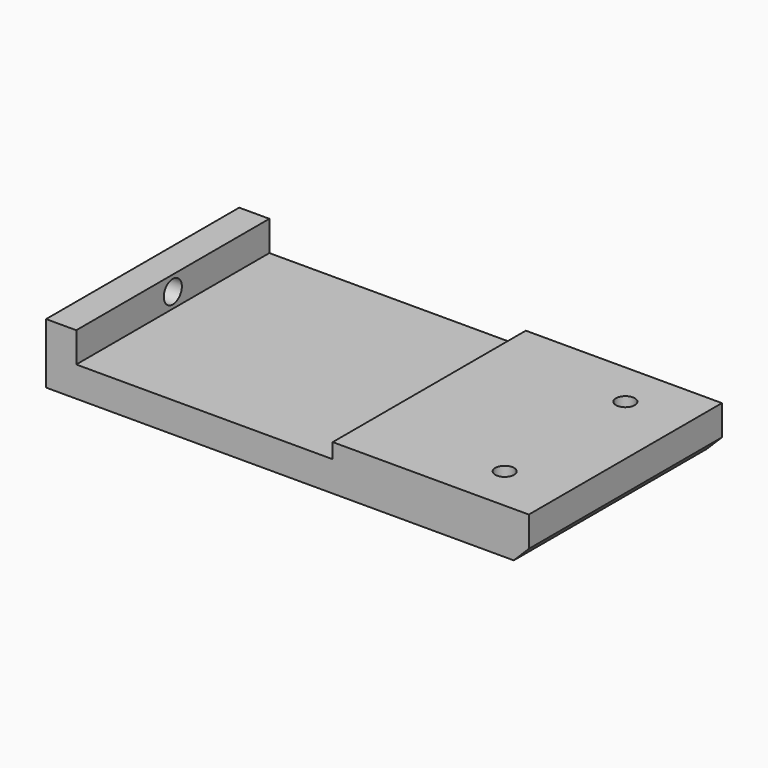
from build123d import *

# Parameters (mm, degrees)
F1_DEPTH = 50.8
F2_SIZE  = 6.35
F4_D     = 7.9375
F6_D     = 9.525
F6_DEPTH = 19.05
F6_TIP   = 2.8615986981


# Not quite as in the source:
# - a length typed as a fraction of an inch, garbled in the dataset ("3 / 203.2 mm" for 3/8 in), is restored


with BuildPart() as f1:
    # F0 (on Front) → F1 (new body, symmetric)
    with BuildSketch(Plane.XZ):
        Polygon((-106.0025989716, 12.7), (-106.0025989716, -12.7), (97.1974010284, -12.7), (97.1974010284, 6.35), (14.6474010284, 6.35), (14.6474010284, 0), (-93.3025989716, 0), (-93.3025989716, 12.7), align=None)
    extrude(amount=F1_DEPTH, both=True)

    # F2
    f2_edges = [f1.edges().sort_by_distance(p)[0] for p in [
        (97.197401, 0, -12.7),
    ]]
    chamfer(f2_edges, length=F2_SIZE)

    # F4 (through all)
    with Locations(Plane.XY.offset(6.35)):
        with Locations((71.7974010284, 31.75), (71.7974010284, -31.75)):
            Hole(F4_D / 2)

    # F6
    with Locations(Plane(origin=(-106.0025989716, 0, 0), x_dir=(0, -1, 0), z_dir=(-1, 0, 0))):
        with Locations((0, 6.35)):
            Hole(F6_D / 2, depth=F6_DEPTH)
            with Locations((0, 0, -(F6_DEPTH + F6_TIP / 2))):  # 118° drill point
                Cone(0, F6_D / 2, F6_TIP, mode=Mode.SUBTRACT)


solid = f1.part
